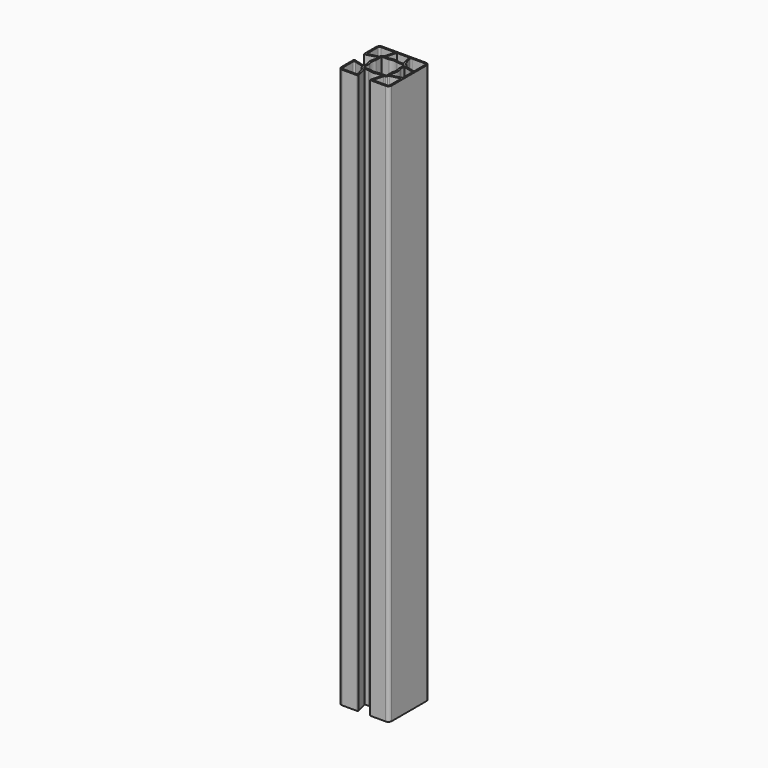
from build123d import *

# Parameters (mm, degrees)
F1_DEPTH = 1000


# Not quite as in the source:
# - ends of sketch curves that miss each other by under 0.0002 mm in the source are joined


with BuildPart() as f1:
    # F0 (on Top) → F1 (new body)
    with BuildSketch(Plane.XY):
        with BuildLine():
            ThreePointArc((8.8614578186, -23.0888885991), (9.062799833, -23.022474706), (9.273618, -23))
            Line((9.273618, -23), (14.841657, -23))
            ThreePointArc((14.841657, -23), (15.6350103133, -23.3912385359), (15.8075828492, -24.2588189596))
            Line((15.8075828492, -24.2588189596), (10.671624, -43.426476))
            ThreePointArc((10.671624, -43.426476), (10.8873403242, -44.5109517857), (11.879032, -45))
            Line((11.879032, -45), (39, -45))
            ThreePointArc((39, -45), (43.2426406871, -43.2426406871), (45, -39))
            Line((45, -39), (45, 39))
            ThreePointArc((45, 39), (43.2426406871, 43.2426406871), (39, 45))
            Line((39, 45), (-39, 45))
            ThreePointArc((-39, 45), (-43.2426406871, 43.2426406871), (-45, 39))
            Line((-45, 39), (-45, 11.879032))
            ThreePointArc((-45, 11.879032), (-44.5109517857, 10.8873403242), (-43.4264761923, 10.6716247175))
            Line((-43.4264761923, 10.6716247175), (-24.258819, 15.807583))
            ThreePointArc((-24.258819, 15.807583), (-23.3912385359, 15.6350103133), (-23, 14.841657))
            Line((-23, 14.841657), (-23, 9.273618))
            ThreePointArc((-23, 9.273618), (-23.022474706, 9.062799833), (-23.0888885991, 8.8614578186))
            ThreePointArc((-23.0888885991, 8.8614578186), (-25, 0), (-23.0888887851, -8.8614579028))
            ThreePointArc((-23.0888887851, -8.8614579028), (-23.022474706, -9.062799833), (-23, -9.273618))
            Line((-23, -9.273618), (-23, -14.841657))
            ThreePointArc((-23, -14.841657), (-23.3912385359, -15.6350103133), (-24.2588189596, -15.8075828492))
            Line((-24.2588189596, -15.8075828492), (-43.426476, -10.671624))
            ThreePointArc((-43.426476, -10.671624), (-44.5109517857, -10.8873403242), (-45, -11.879032))
            Line((-45, -11.879032), (-45, -39))
            ThreePointArc((-45, -39), (-43.2426406871, -43.2426406871), (-39, -45))
            Line((-39, -45), (-11.879032, -45))
            ThreePointArc((-11.879032, -45), (-10.8873403242, -44.5109517857), (-10.6716247175, -43.4264761923))
            Line((-10.6716247175, -43.4264761923), (-15.807583, -24.258819))
            ThreePointArc((-15.807583, -24.258819), (-15.6350103133, -23.3912385359), (-14.841657, -23))
            Line((-14.841657, -23), (-9.273618, -23))
            ThreePointArc((-9.273618, -23), (-9.062799833, -23.022474706), (-8.8614578186, -23.0888885991))
            ThreePointArc((-8.8614578186, -23.0888885991), (0, -25), (8.8614578186, -23.0888885991))
        make_face()
        with BuildLine():
            Line((-39.732362, -14.508469), (-24.482362, -18.594694))
            ThreePointArc((-24.482362, -18.594694), (-23.4132933733, -19.3090230718), (-23, -20.526546))
            Line((-23, -20.526546), (-23, -21))
            ThreePointArc((-23, -21), (-22.4142135624, -22.4142135624), (-21, -23))
            Line((-21, -23), (-20.526546, -23))
            ThreePointArc((-20.526546, -23), (-19.3090230718, -23.4132933733), (-18.5946943016, -24.4823620808))
            Line((-18.5946943016, -24.4823620808), (-14.508469, -39.732362))
            ThreePointArc((-14.508469, -39.732362), (-14.8536143733, -41.4675229282), (-16.440321, -42.25))
            Line((-16.440321, -42.25), (-39, -42.25))
            ThreePointArc((-39, -42.25), (-41.2980970389, -41.2980970389), (-42.25, -39))
            Line((-42.25, -39), (-42.25, -16.440321))
            ThreePointArc((-42.25, -16.440321), (-41.4675229282, -14.8536143733), (-39.732362, -14.508469))
        make_face(mode=Mode.SUBTRACT)
        with BuildLine():
            Line((14.508469, -39.732362), (18.594694, -24.482362))
            ThreePointArc((18.594694, -24.482362), (19.3090230718, -23.4132933733), (20.526546, -23))
            Line((20.526546, -23), (21, -23))
            ThreePointArc((21, -23), (22.4142135624, -22.4142135624), (23, -21))
            Line((23, -21), (23, -20.526546))
            ThreePointArc((23, -20.526546), (23.4132933733, -19.3090230718), (24.4823620808, -18.5946943016))
            Line((24.4823620808, -18.5946943016), (39.732362, -14.508469))
            ThreePointArc((39.732362, -14.508469), (41.4675229282, -14.8536143733), (42.25, -16.440321))
            Line((42.25, -16.440321), (42.25, -39))
            ThreePointArc((42.25, -39), (41.2980970389, -41.2980970389), (39, -42.25))
            Line((39, -42.25), (16.440321, -42.25))
            ThreePointArc((16.440321, -42.25), (14.8536143733, -41.4675229282), (14.508469, -39.732362))
        make_face(mode=Mode.SUBTRACT)
        with BuildLine():
            Line((-7.3951, -20.25), (-19.25, -20.25))
            ThreePointArc((-19.25, -20.25), (-19.9571067812, -19.9571067812), (-20.25, -19.25))
            Line((-20.25, -19.25), (-20.25, -7.3951))
            ThreePointArc((-20.25, -7.3951), (-20.2639867072, -7.2284333074), (-20.3055555728, -7.0664288513))
            ThreePointArc((-20.3055554887, -7.066428822), (-21.5, 0), (-20.3055554887, 7.066428822))
            ThreePointArc((-20.3055555728, 7.0664288513), (-20.2639867072, 7.2284333074), (-20.25, 7.3951))
            Line((-20.25, 7.3951), (-20.25, 19.25))
            ThreePointArc((-20.25, 19.25), (-19.9571067812, 19.9571067812), (-19.25, 20.25))
            Line((-19.25, 20.25), (-7.3951, 20.25))
            ThreePointArc((-7.3951, 20.25), (-7.2284333074, 20.2639867072), (-7.0664288513, 20.3055555728))
            ThreePointArc((-7.066428822, 20.3055554887), (0, 21.5), (7.066428822, 20.3055554887))
            ThreePointArc((7.0664288513, 20.3055555728), (7.2284333074, 20.2639867072), (7.3951, 20.25))
            Line((7.3951, 20.25), (19.25, 20.25))
            ThreePointArc((19.25, 20.25), (19.9571067812, 19.9571067812), (20.25, 19.25))
            Line((20.25, 19.25), (20.25, 7.3951))
            ThreePointArc((20.25, 7.3951), (20.2639867072, 7.2284333074), (20.3055555728, 7.0664288513))
            ThreePointArc((20.3055554887, 7.066428822), (21.5, 0), (20.3055554887, -7.066428822))
            ThreePointArc((20.3055555728, -7.0664288513), (20.2639867072, -7.2284333074), (20.25, -7.3951))
            Line((20.25, -7.3951), (20.25, -19.25))
            ThreePointArc((20.25, -19.25), (19.9571067812, -19.9571067812), (19.25, -20.25))
            Line((19.25, -20.25), (7.3951, -20.25))
            ThreePointArc((7.3951, -20.25), (7.2284333074, -20.2639867072), (7.0664288513, -20.3055555728))
            ThreePointArc((7.066428822, -20.3055554887), (0, -21.5), (-7.066428822, -20.3055554887))
            ThreePointArc((-7.0664288513, -20.3055555728), (-7.2284333074, -20.2639867072), (-7.3951, -20.25))
        make_face(mode=Mode.SUBTRACT)
        with BuildLine():
            Line((42.25, -10.98686), (24.258819, -15.807583))
            ThreePointArc((24.258819, -15.807583), (23.3912385359, -15.6350103133), (23, -14.841657))
            Line((23, -14.841657), (23, -9.273618))
            ThreePointArc((23, -9.273618), (23.022474706, -9.062799833), (23.0888885991, -8.8614578186))
            ThreePointArc((23.0888885991, -8.8614578186), (25, 0), (23.0888887851, 8.8614579028))
            ThreePointArc((23.0888887851, 8.8614579028), (23.022474706, 9.062799833), (23, 9.273618))
            Line((23, 9.273618), (23, 14.841657))
            ThreePointArc((23, 14.841657), (23.3912385359, 15.6350103133), (24.2588189596, 15.8075828492))
            Line((24.2588189596, 15.8075828492), (42.25, 10.98686))
            Line((42.25, 10.98686), (42.25, -10.98686))
        make_face(mode=Mode.SUBTRACT)
        with BuildLine():
            Line((-14.508469, 39.732362), (-18.594694, 24.482362))
            ThreePointArc((-18.594694, 24.482362), (-19.3090230718, 23.4132933733), (-20.526546, 23))
            Line((-20.526546, 23), (-21, 23))
            ThreePointArc((-21, 23), (-22.4142135624, 22.4142135624), (-23, 21))
            Line((-23, 21), (-23, 20.526546))
            ThreePointArc((-23, 20.526546), (-23.4132933733, 19.3090230718), (-24.4823620808, 18.5946943016))
            Line((-24.4823620808, 18.5946943016), (-39.732362, 14.508469))
            ThreePointArc((-39.732362, 14.508469), (-41.4675229282, 14.8536143733), (-42.25, 16.440321))
            Line((-42.25, 16.440321), (-42.25, 39))
            ThreePointArc((-42.25, 39), (-41.2980970389, 41.2980970389), (-39, 42.25))
            Line((-39, 42.25), (-16.440321, 42.25))
            ThreePointArc((-16.440321, 42.25), (-14.8536143733, 41.4675229282), (-14.508469, 39.732362))
        make_face(mode=Mode.SUBTRACT)
        with BuildLine():
            Line((-9.273618, 23), (-14.841657, 23))
            ThreePointArc((-14.841657, 23), (-15.6350103133, 23.3912385359), (-15.8075828492, 24.2588189596))
            Line((-15.8075828492, 24.2588189596), (-10.98686, 42.25))
            Line((-10.98686, 42.25), (10.98686, 42.25))
            Line((10.98686, 42.25), (15.807583, 24.258819))
            ThreePointArc((15.807583, 24.258819), (15.6350103133, 23.3912385359), (14.841657, 23))
            Line((14.841657, 23), (9.273618, 23))
            ThreePointArc((9.273618, 23), (9.062799833, 23.022474706), (8.8614578186, 23.0888885991))
            ThreePointArc((8.8614578186, 23.0888885991), (0, 25), (-8.8614579028, 23.0888887851))
            ThreePointArc((-8.8614579028, 23.0888887851), (-9.062799833, 23.022474706), (-9.273618, 23))
        make_face(mode=Mode.SUBTRACT)
        with BuildLine():
            Line((39.732362, 14.508469), (24.482362, 18.594694))
            ThreePointArc((24.482362, 18.594694), (23.4132933733, 19.3090230718), (23, 20.526546))
            Line((23, 20.526546), (23, 21))
            ThreePointArc((23, 21), (22.4142135624, 22.4142135624), (21, 23))
            Line((21, 23), (20.526546, 23))
            ThreePointArc((20.526546, 23), (19.3090230718, 23.4132933733), (18.5946943016, 24.4823620808))
            Line((18.5946943016, 24.4823620808), (14.508469, 39.732362))
            ThreePointArc((14.508469, 39.732362), (14.8536143733, 41.4675229282), (16.440321, 42.25))
            Line((16.440321, 42.25), (39, 42.25))
            ThreePointArc((39, 42.25), (41.2980970389, 41.2980970389), (42.25, 39))
            Line((42.25, 39), (42.25, 16.440321))
            ThreePointArc((42.25, 16.440321), (41.4675229282, 14.8536143733), (39.732362, 14.508469))
        make_face(mode=Mode.SUBTRACT)
    extrude(amount=F1_DEPTH)


solid = f1.part
